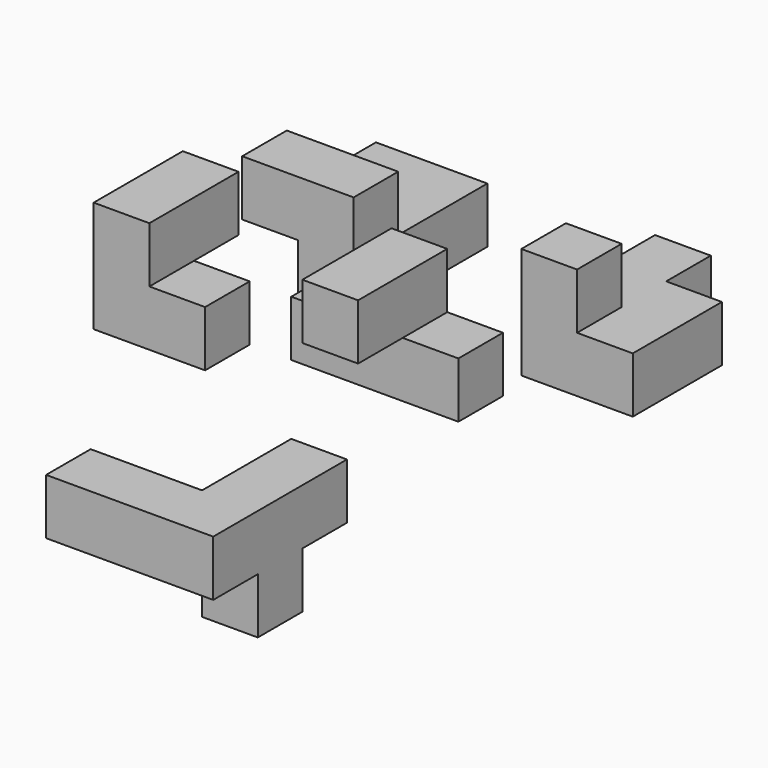
from build123d import *

# Parameters (mm, degrees)
F0_W      = 50.8
F0_H      = 25.4
F1_DEPTH  = 25.4
F2_W      = 25.4
F2_H      = 25.4
F3_DEPTH  = 25.4
F4_W      = 25.4
F4_H      = 25.4
F5_DEPTH  = 25.4
F6_W      = 76.2
F6_H      = 25.4
F7_DEPTH  = 25.4
F8_W      = 25.4
F8_H      = 25.4
F9_DEPTH  = 25.4
F10_W     = 25.4
F10_H     = 25.4
F11_DEPTH = 25.4
F12_W     = 76.2
F12_H     = 25.4
F13_DEPTH = 25.4
F14_W     = 25.4
F14_H     = 25.4
F15_DEPTH = 25.4
F16_W     = 25.4
F16_H     = 25.4
F17_DEPTH = 25.4
F19_W     = 76.2
F19_H     = 25.4
F20_DEPTH = 25.4
F21_W     = 25.3924569011
F21_H     = 25.4
F22_DEPTH = 50.8
F23_W     = 25.4
F23_H     = 25.4037752748
F24_DEPTH = 25.4
F25_W     = 76.2
F25_H     = 25.4
F26_DEPTH = 25.4
F27_W     = 25.4
F27_H     = 25.4
F28_DEPTH = 25.4
F30_DEPTH = 25.4
F32_W     = 76.2
F32_H     = 25.4
F33_DEPTH = 25.4
F34_W     = 25.4
F34_H     = 25.4
F35_DEPTH = 25.4
F36_W     = 25.4
F36_H     = 25.4
F37_DEPTH = 25.4
F38_W     = 25.4
F38_H     = 25.4
F39_DEPTH = 25.4
F41_W     = 25.4
F41_H     = 76.2
F42_DEPTH = 25.4
F43_W     = 25.4
F43_H     = 25.4
F44_DEPTH = 25.4
F45_W     = 25.4
F45_H     = 25.4
F46_DEPTH = 25.4
F47_W     = 25.4
F47_H     = 25.4
F48_DEPTH = 25.4
F49_W     = 50.8
F49_H     = 50.8
F50_DEPTH = 25.4
F51_W     = 25.4
F51_H     = 25.4
F52_DEPTH = 25.4
F53_W     = 25.4
F53_H     = 25.4
F54_DEPTH = 25.4


with BuildPart() as f1:
    # F0 (on Front) → F1 (new body)
    with BuildSketch(Plane.XZ):
        with Locations((-44.3492058954, 12.7)):
            Rectangle(F0_W, F0_H)
    extrude(amount=F1_DEPTH)

    # F2 (on face) → F3 (join)
    with BuildSketch(Plane.XY.offset(25.4)):
        with Locations((-57.0492058954, -12.7)):
            Rectangle(F2_W, F2_H)
    extrude(amount=F3_DEPTH)

    # F4 (on face) → F5 (join)
    with BuildSketch(Plane(origin=(0, 0, 0), x_dir=(-1, 0, 0), z_dir=(0, 1, 0))):
        with Locations((57.0492058954, 38.1)):
            Rectangle(F4_W, F4_H)
    extrude(amount=F5_DEPTH)


with BuildPart() as f7:
    # F6 (on Front) → F7 (new body)
    with BuildSketch(Plane.XZ):
        with Locations((38.1, 12.7)):
            Rectangle(F6_W, F6_H)
    extrude(amount=-F7_DEPTH)

    # F8 (on face) → F9 (join)
    with BuildSketch(Plane.XY.offset(25.4)):
        with Locations((38.1, 12.7)):
            Rectangle(F8_W, F8_H)
    extrude(amount=F9_DEPTH)

    # F10 (on face) → F11 (join)
    with BuildSketch(Plane.XZ):
        with Locations((38.1, 38.1)):
            Rectangle(F10_W, F10_H)
    extrude(amount=F11_DEPTH)


with BuildPart() as f13:
    # F12 (on Front) → F13 (new body)
    with BuildSketch(Plane.XZ):
        with Locations((38.1, -45.3202931168)):
            Rectangle(F12_W, F12_H)
    extrude(amount=F13_DEPTH)

    # F14 (on face) → F15 (join)
    with BuildSketch(Plane(origin=(0, 0, -58.0202931168), x_dir=(1, 0, 0), z_dir=(0, 0, -1))):
        with Locations((38.1, 12.7)):
            Rectangle(F14_W, F14_H)
    extrude(amount=F15_DEPTH)

    # F16 (on face) → F17 (join)
    with BuildSketch(Plane(origin=(0, 0, 0), x_dir=(-1, 0, 0), z_dir=(0, 1, 0))):
        with Locations((-12.7, -45.3202931168)):
            Rectangle(F16_W, F16_H)
    extrude(amount=F17_DEPTH)


with BuildPart() as f20:
    # F19 (on Right) → F20 (new body)
    with BuildSketch(Plane.YZ):
        with Locations((-38.1, -44.3502715829)):
            Rectangle(F19_W, F19_H)
    extrude(amount=F20_DEPTH)

    # F21 (on face) → F22 (join)
    with BuildSketch(Plane(origin=(0, 0, 0), x_dir=(0, -1, 0), z_dir=(-1, 0, 0))):
        with Locations((63.5037715495, -44.3502715829)):
            Rectangle(F21_W, F21_H)
    extrude(amount=F22_DEPTH)

    # F23 (on face) → F24 (join)
    with BuildSketch(Plane(origin=(0, 0, -57.0502715829), x_dir=(1, 0, 0), z_dir=(0, 0, -1))):
        with Locations((12.7, 38.1056554615)):
            Rectangle(F23_W, F23_H)
    extrude(amount=F24_DEPTH)


with BuildPart() as f26:
    # F25 (on Top) → F26 (new body)
    with BuildSketch(Plane.XY):
        with Locations((38.1, -63.4999925264)):
            Rectangle(F25_W, F25_H)
    extrude(amount=F26_DEPTH)

    # F27 (on face) → F28 (join)
    with BuildSketch(Plane(origin=(0, -50.7999925264, 0), x_dir=(-1, 0, 0), z_dir=(0, 1, 0))):
        with Locations((-63.5, 12.7)):
            Rectangle(F27_W, F27_H)
    extrude(amount=F28_DEPTH)

    # F29 (on face) → F30 (join)
    with BuildSketch(Plane.XY.offset(25.4)):
        Polygon((25.4, -76.1999925264), (76.2, -76.1999925264), (76.2, -50.7999925264), (50.8, -50.7999925264), (25.4, -50.7999925264), align=None)
    extrude(amount=F30_DEPTH)


with BuildPart() as f33:
    # F32 (on Top) → F33 (new body)
    with BuildSketch(Plane.XY):
        with Locations((38.1, -63.4999924319)):
            Rectangle(F32_W, F32_H)
    extrude(amount=F33_DEPTH)

    # F34 (on face) → F35 (join)
    with BuildSketch(Plane(origin=(0, -50.7999924319, 0), x_dir=(-1, 0, 0), z_dir=(0, 1, 0))):
        with Locations((-63.5, 12.7)):
            Rectangle(F34_W, F34_H)
    extrude(amount=F35_DEPTH)

    # F36 (on face) → F37 (join)
    with BuildSketch(Plane.XY.offset(25.4)):
        with Locations((12.7, -63.4999924319)):
            Rectangle(F36_W, F36_H)
    extrude(amount=F37_DEPTH)

    # F38 (on face) → F39 (join)
    with BuildSketch(Plane(origin=(0, -50.7999924319, 0), x_dir=(-1, 0, 0), z_dir=(0, 1, 0))):
        with Locations((-12.7, 38.1)):
            Rectangle(F38_W, F38_H)
    extrude(amount=F39_DEPTH)


with BuildPart() as f42:
    # F41 (on Top) → F42 (new body)
    with BuildSketch(Plane.XY):
        with Locations((-12.7, 73.6599986479)):
            Rectangle(F41_W, F41_H)
    extrude(amount=F42_DEPTH)

    # F43 (on face) → F44 (join)
    with BuildSketch(Plane.XY.offset(25.4)):
        with Locations((-12.7, 48.2599986479)):
            Rectangle(F43_W, F43_H)
    extrude(amount=F44_DEPTH)

    # F45 (on face) → F46 (join)
    with BuildSketch(Plane(origin=(-25.4, 0, 0), x_dir=(0, -1, 0), z_dir=(-1, 0, 0))):
        with Locations((-48.2599986479, 38.1)):
            Rectangle(F45_W, F45_H)
    extrude(amount=F46_DEPTH)

    # F47 (on face) → F48 (join)
    with BuildSketch(Plane(origin=(-25.4, 0, 0), x_dir=(0, -1, 0), z_dir=(-1, 0, 0))):
        with Locations((-99.0599986479, 12.7)):
            Rectangle(F47_W, F47_H)
    extrude(amount=F48_DEPTH)


with BuildPart() as f50:
    # F49 (on Top) → F50 (new body)
    with BuildSketch(Plane.XY):
        with Locations((96.8366935334, 67.232016474)):
            Rectangle(F49_W, F49_H)
    extrude(amount=F50_DEPTH)

    # F51 (on face) → F52 (join)
    with BuildSketch(Plane.XY.offset(25.4)):
        with Locations((84.1366935334, 54.532016474)):
            Rectangle(F51_W, F51_H)
    extrude(amount=F52_DEPTH)

    # F53 (on face) → F54 (join)
    with BuildSketch(Plane(origin=(0, 92.632016474, 0), x_dir=(-1, 0, 0), z_dir=(0, 1, 0))):
        with Locations((-84.1366935334, 12.7)):
            Rectangle(F53_W, F53_H)
    extrude(amount=F54_DEPTH)


solid = Compound([f1.part, f7.part, f20.part, f42.part, f50.part])
